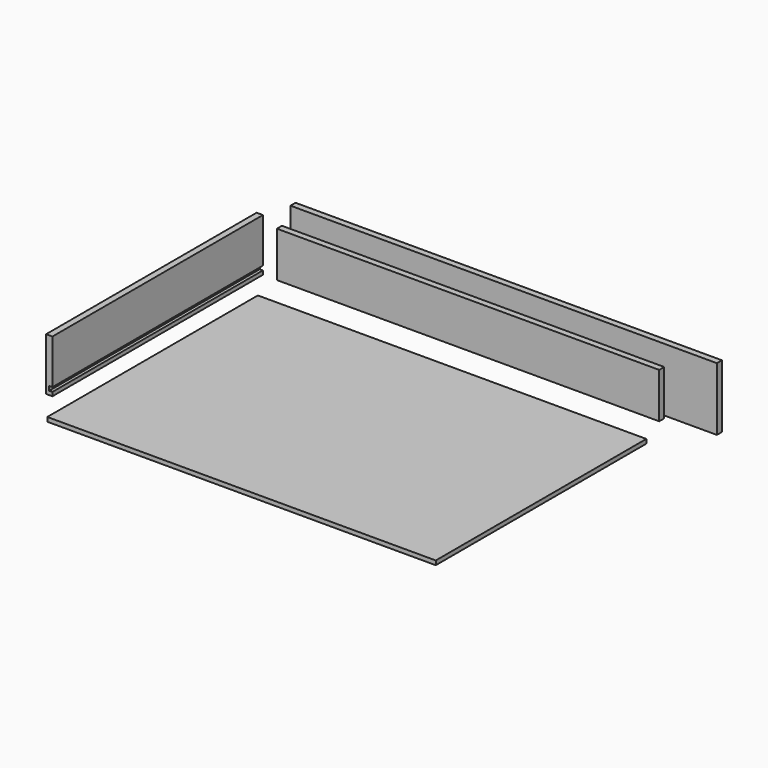
from build123d import *

# Parameters (mm, degrees)
F1_DEPTH = 500
F2_W     = 738
F2_H     = 8
F3_DEPTH = 500
F4_W     = 12
F4_H     = 86
F5_DEPTH = 726.4
F6_W     = 12
F6_H     = 120
F7_DEPTH = 810


# Not quite as in the source:
# - a feature names something its author has since deleted; it is built from what else it names


with BuildPart() as f1:
    # F0 (on Front) → F1 (new body)
    with BuildSketch(Plane.XZ):
        Polygon((-1.8907085117, 77.3167183763), (-13.8907085117, 77.3167183763), (-13.8907085117, -22.6832816237), (-1.8907085117, -22.6832816237), (-1.8907085117, -15.298666623), (-7.8907085117, -15.298666623), (-7.8907085117, -7.298666623), (-1.8907085117, -7.298666623), align=None)
    extrude(amount=F1_DEPTH)


with BuildPart() as f3:
    # F2 (on Front) → F3 (new body)
    with BuildSketch(Plane.XZ):
        with Locations((357.4027951019, -64.3239161)):
            Rectangle(F2_W, F2_H)
    extrude(amount=F3_DEPTH)


with BuildPart() as f5:
    # F4 (on Right) → F5 (new body)
    with BuildSketch(Plane.YZ):
        with Locations((36.6045031697, -0.3242592409)):
            Rectangle(F4_W, F4_H)
    extrude(amount=F5_DEPTH)


with BuildPart() as f7:
    # F6 (on Right) → F7 (new body)
    with BuildSketch(Plane.YZ):
        with Locations((69.0702423453, 7.9040200152)):
            Rectangle(F6_W, F6_H)
    extrude(amount=F7_DEPTH)


solid = Compound([f1.part, f3.part, f5.part, f7.part])
